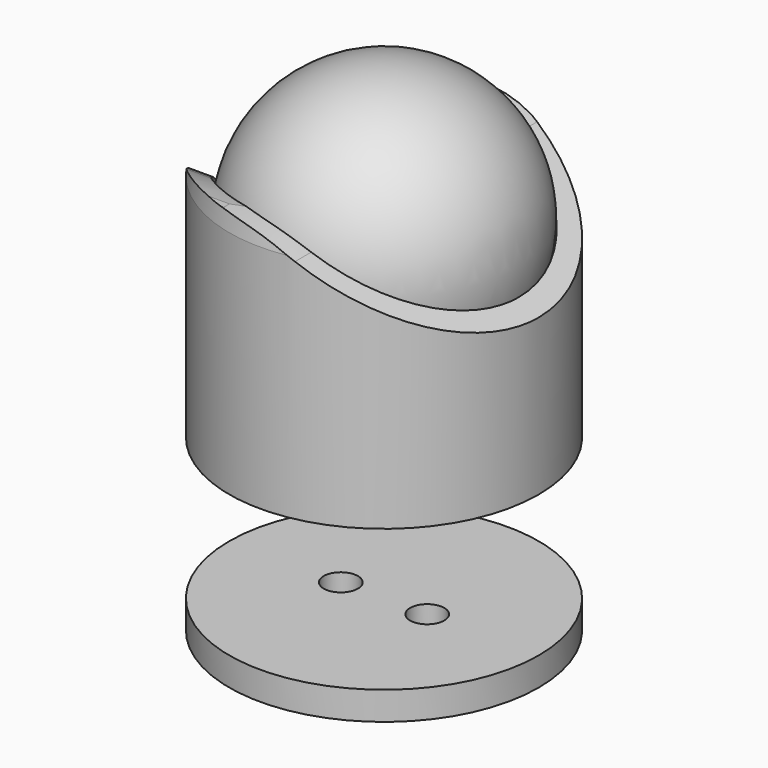
from build123d import *

# Parameters (mm, degrees)
F0_R      = 10.922
F0_R_2    = 1.2065
F1_DEPTH  = 17.4
F3_SIZE2  = 1.1342563639
F3_SIZE   = 0.2
F4_DEPTH  = 12.5
F7_R      = 9.522
F8_DEPTH  = 15
F10_DEPTH = 25
F15_R     = 10.922
F15_R_2   = 1.2065
F16_DEPTH = 2


# Not quite as in the source:
# - the dataset's text gives a spline's control points without its knots; the knots are read off the source's solid


with BuildPart() as f1:
    # F0 (on Top) → F1 (new body)
    with BuildSketch(Plane.XY):
        Circle(F0_R)
        with Locations((-3.048, 0)):
            Circle(F0_R_2, mode=Mode.SUBTRACT)
        with Locations((3.048, 0)):
            Circle(F0_R_2, mode=Mode.SUBTRACT)
    extrude(amount=F1_DEPTH)

    # F3
    f3_edges = [f1.edges().sort_by_distance(p)[0] for p in [
        (-10.922, 0, 17.4),
    ]]
    f3_side = f1.faces().sort_by_distance((0, 0, 17.4))[0]
    chamfer(f3_edges, length=F3_SIZE, length2=F3_SIZE2, reference=f3_side)

    # F2 (on Front) → F4 (intersect, symmetric)
    with BuildSketch(Plane.XZ):
        with BuildLine():
            Line((-10.922, 2.5240874384), (-10.922, 0))
            Line((-10.922, 0), (10.922, 0))
            Line((10.922, 0), (10.922, 11))
            Line((10.922, 11), (2.2617459622, 16))
            add(Edge.make_bspline(
                [(-10.5561679229, 12.3512884602), (-10.5561679229, 13.3744198827), (-10.3092380287, 15.4668604941), (-7.3744263519, 17.5564003065), (-0.8273779191, 17.4793571937), (1.3828107736, 16.5074534677), (2.2617459622, 16)],
                knots=[0, 0, 0, 0, 0.2167373825, 0.4454441549, 0.7666030159, 1, 1, 1, 1], degree=3))
            Line((-10.5561679229, 12.3512884602), (-10.5561679229, 5.1718307659))
            add(Edge.make_bspline(
                [(-10.922, 2.5240874384), (-10.8079449165, 2.922149178), (-10.5748505542, 3.7446575215), (-10.5561679229, 4.6860097011), (-10.5561679229, 5.1718307659)],
                knots=[0, 0, 0, 0, 0.4839692719, 1, 1, 1, 1], degree=3))
        make_face()
    extrude(amount=F4_DEPTH, both=True, mode=Mode.INTERSECT)

    # F7 (on plane+point) → F8 (cut)
    with BuildSketch(Plane.XY.offset(17.4)):
        Circle(F7_R)
    extrude(amount=-F8_DEPTH, mode=Mode.SUBTRACT)

    # F9 (on Right) → F10 (cut)
    with BuildSketch(Plane.YZ):
        with BuildLine():
            add(Edge.make_bspline(
                [(-6.1908482033, 16.2657436361), (-5.8239832679, 16.0842065539), (-5.2697423367, 15.7782810678), (-4.5449625596, 15.2817000949), (-4.0150312361, 14.8437308416), (-3.530892932, 14.3383630089), (-3.1908678442, 13.8451050056), (-2.9903637846, 13.4152056187), (-2.8421915125, 12.9531733158), (-2.8031059172, 12.5940113653), (-2.8031059172, 12.3512884602)],
                knots=[0, 0, 0, 0, 0.001422398, 0.002133597, 0.002844796, 0.003555995, 0.004267194, 0.0046227935, 0.004978393, 0.005689592, 0.005689592, 0.005689592, 0.005689592], degree=3))
            Line((-2.8031059172, 12.3512884602), (-2.8031059172, 5.1718307659))
            add(Edge.make_bspline(
                [(-2.8031059172, 5.1718307659), (-2.8031059172, 4.9880839005), (-2.7931824983, 4.620933965), (-2.7035715856, 4.1692868315), (-2.5590327547, 3.8361950373), (-2.4079078984, 3.6051620635), (-2.2282574542, 3.4038210692), (-1.9542751637, 3.1613240966), (-1.5776780577, 2.9167479541), (-1.0741099879, 2.6946871782), (-0.549175924, 2.556618218), (0.0034570563, 2.5080192737), (0.5439942396, 2.5558313081), (1.0786692315, 2.6962222432), (1.5737683379, 2.9145895187), (1.9576551695, 3.1640660292), (2.2271837234, 3.4027000426), (2.4101315065, 3.6080646978), (2.5580933005, 3.8346759648), (2.6681186157, 4.0876015562), (2.7400377264, 4.3519615447), (2.7953024448, 4.7115969912), (2.8031059172, 4.988205093), (2.8031059172, 5.1718307659)],
                knots=[0, 0, 0, 0, 0.0005499451, 0.0010998902, 0.0013748627, 0.0016498353, 0.0019248078, 0.0021997803, 0.0027497254, 0.0032996705, 0.0038496156, 0.0043995607, 0.0049495058, 0.0054994509, 0.006049396, 0.006599341, 0.0068743136, 0.0071492861, 0.0074242587, 0.0076992312, 0.0079742038, 0.0082491763, 0.0087991214, 0.0087991214, 0.0087991214, 0.0087991214], degree=3))
            Line((2.8031059172, 5.1718307659), (2.8031059172, 12.3512884602))
            add(Edge.make_bspline(
                [(2.8031059172, 12.3512884602), (2.8031059172, 12.5934425958), (2.8416241837, 12.9484715212), (2.9877267243, 13.4087416016), (3.1388073995, 13.7338683343), (3.3225041635, 14.0363380259), (3.6071181437, 14.4172462357), (4.0069233774, 14.8358898672), (4.5325996334, 15.2726243288), (5.2687163212, 15.7783118456), (5.8238362153, 16.0841337873), (6.1908482033, 16.2657436361)],
                knots=[0, 0, 0, 0, 0.0007152017, 0.0010728026, 0.0014304035, 0.0017880044, 0.0021456052, 0.002860807, 0.0035760087, 0.0042912105, 0.005721614, 0.005721614, 0.005721614, 0.005721614], degree=3))
            add(Edge.make_bspline(
                [(9.6622267155, 17.4), (9.4555061994, 17.3823981242), (8.993583202, 17.3156789778), (8.1658745172, 17.1195865927), (7.2099218751, 16.7899386077), (6.5331166458, 16.4659237452), (6.1908482033, 16.2657436361)],
                knots=[0, 0, 0, 0, 0.0014302791, 0.0028605583, 0.0042908374, 0.0057211165, 0.0057211165, 0.0057211165, 0.0057211165], degree=3))
            Line((9.6622267155, 17.4), (-9.6622267155, 17.4))
            add(Edge.make_bspline(
                [(-6.1908482033, 16.2657436361), (-6.533077676, 16.4659009532), (-7.2079421108, 16.7885296422), (-7.9953825417, 17.0616275711), (-8.5760965596, 17.2162609075), (-9.108415903, 17.3326312008), (-9.4556098256, 17.3824069477), (-9.6622267155, 17.4)],
                knots=[0, 0, 0, 0, 0.0014325311, 0.0028650621, 0.0035813276, 0.0042975932, 0.0057301242, 0.0057301242, 0.0057301242, 0.0057301242], degree=3))
        make_face()
    extrude(amount=-F10_DEPTH, mode=Mode.SUBTRACT)


with BuildPart() as f13:
    # F12 (on offset) → F13 (revolve)
    with BuildSketch(Plane.XY.offset(13.61)):
        with BuildLine():
            ThreePointArc((0, -9.5), (9.5, 0), (0, 9.5))
            Line((0, 9.5), (0, -9.5))
        make_face()
    revolve(axis=Axis((0, 0, 13.61), (0, -1, 0)))


with BuildPart() as f16:
    # F15 (on offset) → F16 (new body)
    with BuildSketch(Plane(origin=(0, 0, -10), x_dir=(1, 0, 0), z_dir=(0, 0, -1))):
        Circle(F15_R)
        with Locations((-3.048, 0)):
            Circle(F15_R_2, mode=Mode.SUBTRACT)
        with Locations((3.048, 0)):
            Circle(F15_R_2, mode=Mode.SUBTRACT)
    extrude(amount=F16_DEPTH)


solid = Compound([f1.part, f13.part, f16.part])
